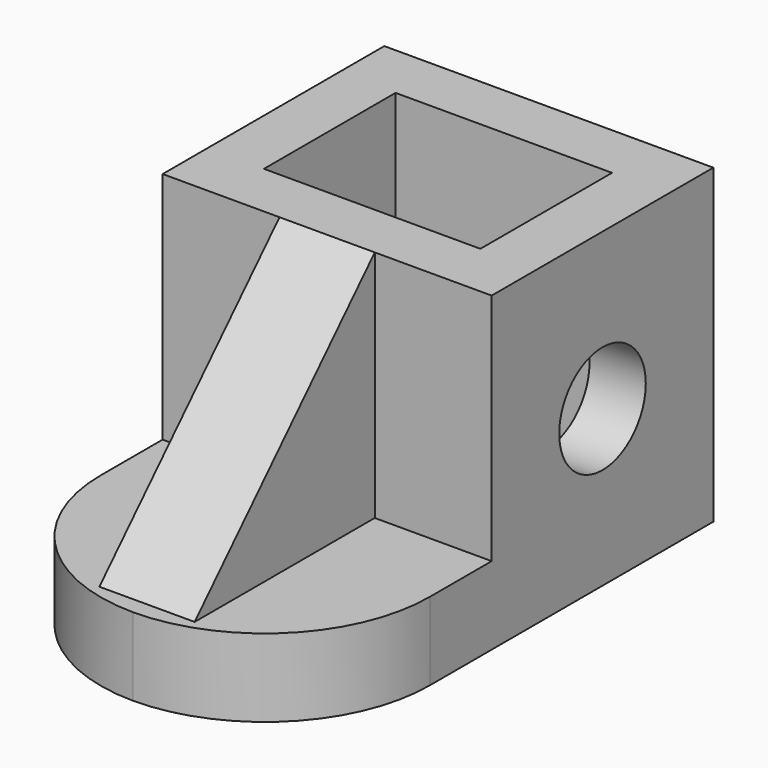
from build123d import *

# Parameters (mm, degrees)
F2_DEPTH    = 76
F3_R        = 12.5
F4_DEPTH    = 127.1
F6_DEPTH    = 53.4
F7_T1_DEPTH = 208.7228714275
F8_W        = 11
F8_H        = 54
F9_DEPTH    = 52
F10_W       = 11
F10_H       = 54
F11_DEPTH   = 52
F13_DEPTH   = 67.9
F14_W       = 50
F14_H       = 38
F15_DEPTH   = 79.6


# Not quite as in the source:
# - a fillet or chamfer that OpenCascade refuses, or shapes differently, is made with other operations: its cross-section is extruded or revolved along the edge and cut away or added


with BuildPart() as f2:
    # F1 (on Right) → F2 (new body)
    with BuildSketch(Plane.YZ):
        Polygon((-74.8220309615, 18), (-74.8220309615, 0), (45.1779690385, 0), (45.1779690385, 72), (-18.8220309615, 72), (-18.8220309615, 18), align=None)
    extrude(amount=F2_DEPTH)

    # F3 (on face) → F4 (cut)
    with BuildSketch(Plane.YZ.offset(76)):
        with Locations((13.1779690385, 36)):
            Circle(F3_R)
    extrude(amount=-F4_DEPTH, mode=Mode.SUBTRACT)

    # F5 (on face) → F6 (cut)
    with BuildSketch(Plane.XY.offset(72)):
        Polygon((13, 32.1779690385), (13, 13.1779690385), (13, -5.8220309615), (28.5150296986, -5.8220309615), (63, -5.8220309615), (63, 16.2556339055), (63, 32.1779690385), (35.4323200881, 32.1779690385), align=None)
    extrude(amount=-F6_DEPTH, mode=Mode.SUBTRACT)

    # F7: fillet of radius 38.1445742855 on 2 edges, made by hand

    # F7_s2 → F7_t1 (cut)
    with BuildSketch(Plane.XY.offset(-95.3614357137)):
        with BuildLine():
            ThreePointArc((38.1445742855, -74.8220309615), (11.1722871427, -63.6497438188), (0, -36.677456676))
            Line((0, -36.677456676), (0, -74.8220309615))
            Line((0, -74.8220309615), (38.1445742855, -74.8220309615))
        make_face()
        with BuildLine():
            ThreePointArc((37.8554257145, -74.8220309615), (64.8277128573, -63.6497438188), (76, -36.677456676))
            Line((76, -36.677456676), (76, -74.8220309615))
            Line((76, -74.8220309615), (37.8554257145, -74.8220309615))
        make_face()
    extrude(amount=F7_T1_DEPTH, mode=Mode.SUBTRACT)

    # F8 (on face) → F9 (join)
    with BuildSketch(Plane.XZ.offset(18.8220309615)):
        with Locations((32.5, 45)):
            Rectangle(F8_W, F8_H)
    extrude(amount=F9_DEPTH)

    # F10 (on face) → F11 (join)
    with BuildSketch(Plane.XZ.offset(18.8220309615)):
        with Locations((43.5, 45)):
            Rectangle(F10_W, F10_H)
    extrude(amount=F11_DEPTH)

    # F12 (on face) → F13 (cut)
    with BuildSketch(Plane.YZ.offset(49)):
        Polygon((-70.8220309615, 72), (-70.8220309615, 18), (-18.8220309615, 72), align=None)
    extrude(amount=-F13_DEPTH, mode=Mode.SUBTRACT)

    # F14 (on face) → F15 (cut)
    with BuildSketch(Plane.XY.offset(18.6)):
        with Locations((38, 13.1779690385)):
            Rectangle(F14_W, F14_H)
    extrude(amount=-F15_DEPTH, mode=Mode.SUBTRACT)


solid = f2.part
